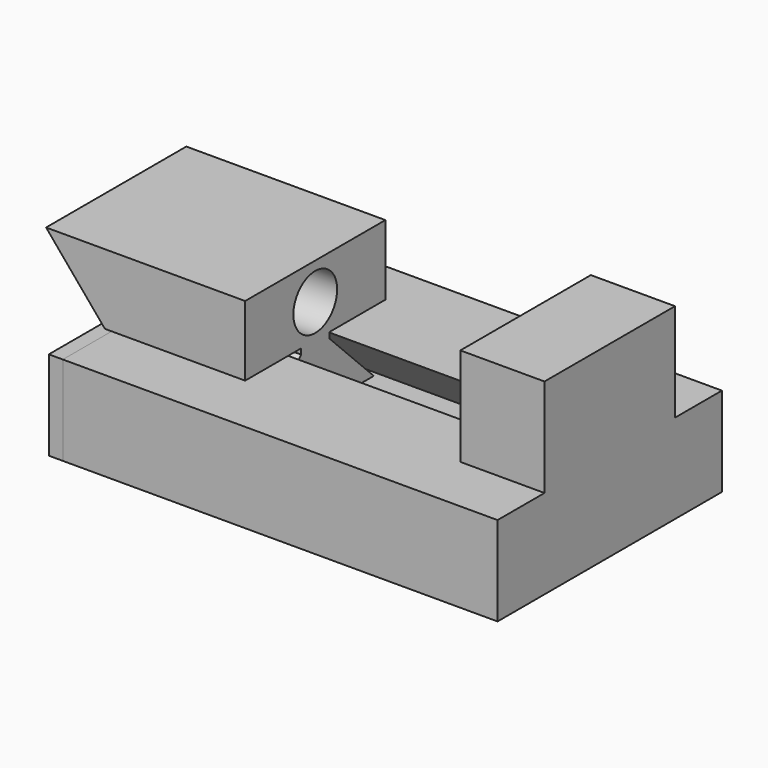
from build123d import *

# Parameters (mm, degrees)
F2_DEPTH  = 25
F3_DEPTH  = 10
F5_DEPTH  = 12.5
F7_DEPTH  = 6
F9_DEPTH  = 7
F11_DEPTH = 3
F12_R     = 1.95
F12_R_2   = 1
F13_DEPTH = 3
F15_DEPTH = 1


# Not quite as in the source:
# - a feature names something its author has since deleted; it is built from what else it names


with BuildPart() as f2:
    # F1 (on Right) → F2 (new body)
    with BuildSketch(Plane.YZ):
        Polygon((10, -6.3646009103), (10, 0), (1.8156854249, 0), (6.1802863352, -4.3646009103), (0, -4.3646009103), (-6.1802863352, -4.3646009103), (-1.8156854249, 0), (-10, 0), (-10, -6.3646009103), (0, -6.3646009103), align=None)
    extrude(amount=F2_DEPTH)

    # F6 (on face) → F7 (join)
    with BuildSketch(Plane.YZ.offset(25)):
        Polygon((-6.1802863352, -4.3646009103), (-1.8156854249, 0), (-10, 0), (-10, -6.3646009103), (10, -6.3646009103), (10, 0), (1.8156854249, 0), (6.1802863352, -4.3646009103), align=None)
        Polygon((1.8156854249, 0), (-1.8156854249, 0), (-6.1802863352, -4.3646009103), (6.1802863352, -4.3646009103), align=None)
    extrude(amount=F7_DEPTH)

    # F8 (on face) → F9 (join)
    with BuildSketch(Plane.XY):
        Polygon((25, 1.8156854249), (25, -1.8156854249), (25, -5.8156854249), (31, -5.8156854249), (31, 5.8156854249), (25, 5.8156854249), align=None)
    extrude(amount=F9_DEPTH)

    # F10 (on face) → F11 (cut)
    with BuildSketch(Plane(origin=(25, 0, 0), x_dir=(0, -1, 0), z_dir=(-1, 0, 0))):
        with BuildLine():
            ThreePointArc((1.1456439237, 5.4), (0, 5.65), (-1.1456439237, 5.4))
            Line((-1.1456439237, 5.4), (1.1456439237, 5.4))
        make_face()
        with BuildLine():
            Line((1.1456439237, 5.4), (-1.1456439237, 5.4))
            ThreePointArc((-1.1456439237, 5.4), (-1.4852574204, 0.585586382), (2.75, 2.9))
            ThreePointArc((2.75, 2.9), (2.314413618, 4.3852574204), (1.1456439237, 5.4))
        make_face()
    extrude(amount=-F11_DEPTH, mode=Mode.SUBTRACT)


with BuildPart() as f3:
    # F1 (on Right) → F3 (new body)
    with BuildSketch(Plane.YZ):
        Polygon((0, -3.9646009103), (5.2146009103, -3.9646009103), (1.25, 0), (1.25, 0.4), (6.25, 0.4), (6.25, 5.4), (0, 5.4), (-6.25, 5.4), (-6.25, 0.4), (-1.25, 0.4), (-1.25, 0), (-5.2146009103, -3.9646009103), align=None)
    extrude(amount=F3_DEPTH)

    # F4 (on face) → F5 (join, through all)
    with BuildSketch(Plane.XZ.offset(6.25)):
        Polygon((-4.1954981559, 5.4), (0, 0.4), (0, 5.4), align=None)
    extrude(amount=-F5_DEPTH)

    # F12 (on face) → F13 (cut)
    with BuildSketch(Plane.YZ.offset(10)):
        with Locations((0, 2.8)):
            Circle(F12_R)
        with Locations((0, 2.8)):
            Circle(F12_R_2, mode=Mode.SUBTRACT)
        with Locations((0, 2.8)):
            Circle(F12_R_2)
    extrude(amount=-F13_DEPTH, mode=Mode.SUBTRACT)


with BuildPart() as f15:
    # F14 (on face) → F15 (new body)
    with BuildSketch(Plane.YZ):
        Polygon((0.1802863352, -0.3646009103), (4.1802863352, -0.3646009103), (4.1802863352, 0), (-10, 0), (-10, -6.3646009103), (0, -6.3646009103), (10, -6.3646009103), (10, -2), (6, -2), (6, -4.3646009103), (0.1802863352, -4.3646009103), align=None)
        Polygon((4.1802863352, 0), (4.1802863352, -0.3646009103), (0.1802863352, -0.3646009103), (0.1802863352, -4.3646009103), (6, -4.3646009103), (6, -2), (10, -2), (10, 0), align=None)
    extrude(amount=-F15_DEPTH)


solid = Compound([f2.part, f3.part, f15.part])
